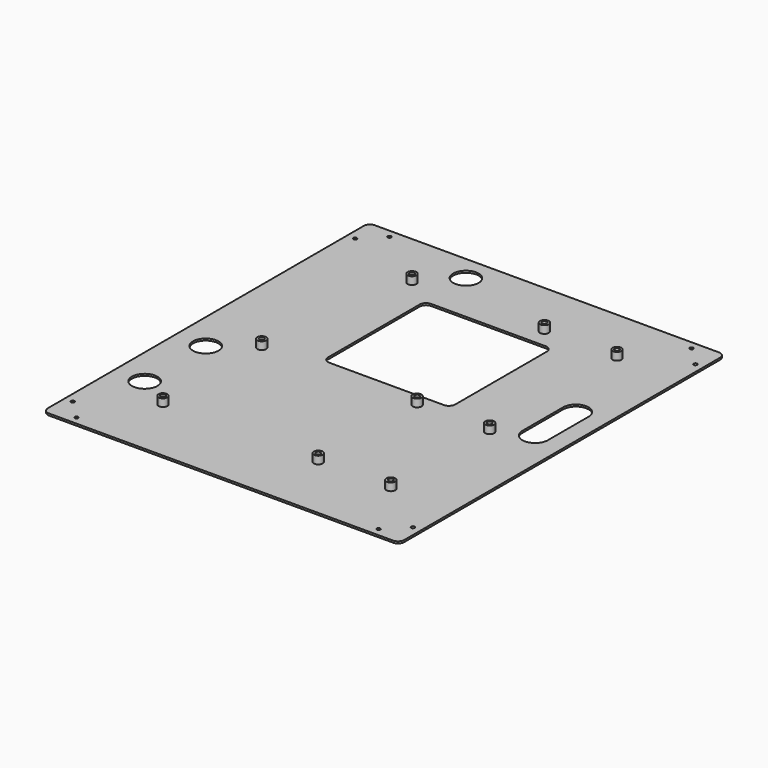
from build123d import *

# Parameters (mm, degrees)
F0_R     = 1.7526
F0_R_2   = 12.7
F0_R_3   = 4.445
F1_DEPTH = 1.905
F0_R_4   = 2.3876
F2_DEPTH = 9.525


# Not quite as in the source:
# - a feature names something its author has since deleted; it is built from what else it names


with BuildPart() as f1:
    # F0 (on Top) → F1 (new body)
    with BuildSketch(Plane.XY):
        with BuildLine():
            Line((192.8597838237, 278.8835931593), (-150.0402161763, 278.8835931593))
            ThreePointArc((-150.0402161763, 278.8835931593), (-154.5303442368, 277.0237212199), (-156.3902161763, 272.5335931593))
            Line((-156.3902161763, 272.5335931593), (-156.3902161763, -121.1664068407))
            ThreePointArc((-156.3902161763, -121.1664068407), (-154.5303442368, -125.6565349012), (-150.0402161763, -127.5164068407))
            Line((-150.0402161763, -127.5164068407), (192.8597838237, -127.5164068407))
            ThreePointArc((192.8597838237, -127.5164068407), (197.3499118843, -125.6565349012), (199.2097838237, -121.1664068407))
            Line((199.2097838237, -121.1664068407), (199.2097838237, 272.5335931593))
            ThreePointArc((199.2097838237, 272.5335931593), (197.3499118843, 277.0237212199), (192.8597838237, 278.8835931593))
        make_face()
        with Locations((-129.2376161763, -119.4138068407)):
            Circle(F0_R, mode=Mode.SUBTRACT)
        with Locations((-148.2876161763, -100.3638068407)):
            Circle(F0_R, mode=Mode.SUBTRACT)
        with Locations((-125.9102161763, -38.6164068407)):
            Circle(F0_R_2, mode=Mode.SUBTRACT)
        with Locations((-125.9102161763, 37.5835931593)):
            Circle(F0_R_2, mode=Mode.SUBTRACT)
        with Locations((172.0571838237, -119.4138068407)):
            Circle(F0_R, mode=Mode.SUBTRACT)
        with Locations((191.1071838237, -100.3638068407)):
            Circle(F0_R, mode=Mode.SUBTRACT)
        with Locations((-148.2876161763, 251.7309931593)):
            Circle(F0_R, mode=Mode.SUBTRACT)
        with Locations((-129.2376161763, 270.7809931593)):
            Circle(F0_R, mode=Mode.SUBTRACT)
        with Locations((-39.1178902483, 253.4835931593)):
            Circle(F0_R_2, mode=Mode.SUBTRACT)
        Polygon((64.5897838237, -76.7164068407), (-100.5102161763, -76.7164068407), (-100.5102161763, 140.7156608748), (-100.5102161763, 228.0835931593), (143.3297838237, 228.0835931593), (143.3297838237, -76.7164068407), align=None, mode=Mode.SUBTRACT)
        with BuildLine():
            Line((156.0297838237, 79.9791118101), (156.0297838237, 130.7791118101))
            ThreePointArc((156.0297838237, 130.7791118101), (168.7297838237, 143.4791118101), (181.4297838237, 130.7791118101))
            Line((181.4297838237, 130.7791118101), (181.4297838237, 79.9791118101))
            ThreePointArc((181.4297838237, 79.9791118101), (168.7297838237, 67.2791118101), (156.0297838237, 79.9791118101))
        make_face(mode=Mode.SUBTRACT)
        with Locations((191.1071838237, 251.7309931593)):
            Circle(F0_R, mode=Mode.SUBTRACT)
        with Locations((172.0571838237, 270.7809931593)):
            Circle(F0_R, mode=Mode.SUBTRACT)
        Polygon((-100.5102161763, 140.7156608748), (-100.5102161763, -76.7164068407), (64.5897838237, -76.7164068407), (143.3297838237, -76.7164068407), (143.3297838237, 228.0835931593), (-100.5102161763, 228.0835931593), align=None)
        with Locations((-90.3502161763, -60.2064068407)):
            Circle(F0_R_3, mode=Mode.SUBTRACT)
        with Locations((-90.3502161763, 62.9835931593)):
            Circle(F0_R_3, mode=Mode.SUBTRACT)
        with Locations((64.5897838237, -60.2064068407)):
            Circle(F0_R_3, mode=Mode.SUBTRACT)
        with Locations((136.9797838237, -60.2064068407)):
            Circle(F0_R_3, mode=Mode.SUBTRACT)
        with Locations((64.5897838237, 62.9835931593)):
            Circle(F0_R_3, mode=Mode.SUBTRACT)
        with Locations((136.9797838237, 62.9835931593)):
            Circle(F0_R_3, mode=Mode.SUBTRACT)
        with Locations((-67.4902161763, 221.7335931593)):
            Circle(F0_R_3, mode=Mode.SUBTRACT)
        with BuildLine():
            Line((-33.2002161763, 202.6835931593), (81.0997838237, 202.6835931593))
            ThreePointArc((81.0997838237, 202.6835931593), (85.5899118843, 200.8237212199), (87.4497838237, 196.3335931593))
            Line((87.4497838237, 196.3335931593), (87.4497838237, 82.0335931593))
            ThreePointArc((87.4497838237, 82.0335931593), (85.5899118843, 77.5434650988), (81.0997838237, 75.6835931593))
            Line((81.0997838237, 75.6835931593), (-33.2002161763, 75.6835931593))
            ThreePointArc((-33.2002161763, 75.6835931593), (-37.6903442368, 77.5434650988), (-39.5502161763, 82.0335931593))
            Line((-39.5502161763, 82.0335931593), (-39.5502161763, 196.3335931593))
            ThreePointArc((-39.5502161763, 196.3335931593), (-37.6903442368, 200.8237212199), (-33.2002161763, 202.6835931593))
        make_face(mode=Mode.SUBTRACT)
        with Locations((64.5897838237, 221.7335931593)):
            Circle(F0_R_3, mode=Mode.SUBTRACT)
        with Locations((136.9797838237, 221.7335931593)):
            Circle(F0_R_3, mode=Mode.SUBTRACT)
    extrude(amount=F1_DEPTH)


with BuildPart() as f1b:
    # F0 (on Top) → F1, piece 2 (new body)
    with BuildSketch(Plane.XY):
        with Locations((64.5897838237, 62.9835931593)):
            Circle(F0_R_4)
    extrude(amount=F1_DEPTH)


with BuildPart() as f1c:
    # F0 (on Top) → F1, piece 3 (new body)
    with BuildSketch(Plane.XY):
        with Locations((-90.3502161763, 62.9835931593)):
            Circle(F0_R_4)
    extrude(amount=F1_DEPTH)


with BuildPart() as f1d:
    # F0 (on Top) → F1, piece 4 (new body)
    with BuildSketch(Plane.XY):
        with Locations((-90.3502161763, -60.2064068407)):
            Circle(F0_R_4)
    extrude(amount=F1_DEPTH)


with BuildPart() as f1e:
    # F0 (on Top) → F1, piece 5 (new body)
    with BuildSketch(Plane.XY):
        with Locations((64.5897838237, -60.2064068407)):
            Circle(F0_R_4)
    extrude(amount=F1_DEPTH)


with BuildPart() as f1f:
    # F0 (on Top) → F1, piece 6 (new body)
    with BuildSketch(Plane.XY):
        with Locations((136.9797838237, -60.2064068407)):
            Circle(F0_R_4)
    extrude(amount=F1_DEPTH)


with BuildPart() as f2:
    # F0 (on Top) → F2 (new body)
    with BuildSketch(Plane.XY):
        with Locations((-90.3502161763, -60.2064068407)):
            Circle(F0_R_3)
        with Locations((-90.3502161763, -60.2064068407)):
            Circle(F0_R_4, mode=Mode.SUBTRACT)
    extrude(amount=F2_DEPTH)


with BuildPart() as f2b:
    # F0 (on Top) → F2, piece 2 (new body)
    with BuildSketch(Plane.XY):
        with Locations((-90.3502161763, 62.9835931593)):
            Circle(F0_R_3)
        with Locations((-90.3502161763, 62.9835931593)):
            Circle(F0_R_4, mode=Mode.SUBTRACT)
    extrude(amount=F2_DEPTH)


with BuildPart() as f2c:
    # F0 (on Top) → F2, piece 3 (new body)
    with BuildSketch(Plane.XY):
        with Locations((64.5897838237, 62.9835931593)):
            Circle(F0_R_3)
        with Locations((64.5897838237, 62.9835931593)):
            Circle(F0_R_4, mode=Mode.SUBTRACT)
    extrude(amount=F2_DEPTH)


with BuildPart() as f2d:
    # F0 (on Top) → F2, piece 4 (new body)
    with BuildSketch(Plane.XY):
        with Locations((136.9797838237, 62.9835931593)):
            Circle(F0_R_3)
        with Locations((136.9797838237, 62.9835931593)):
            Circle(F0_R_4, mode=Mode.SUBTRACT)
    extrude(amount=F2_DEPTH)


with BuildPart() as f2e:
    # F0 (on Top) → F2, piece 5 (new body)
    with BuildSketch(Plane.XY):
        with Locations((64.5897838237, -60.2064068407)):
            Circle(F0_R_3)
        with Locations((64.5897838237, -60.2064068407)):
            Circle(F0_R_4, mode=Mode.SUBTRACT)
    extrude(amount=F2_DEPTH)


with BuildPart() as f2f:
    # F0 (on Top) → F2, piece 6 (new body)
    with BuildSketch(Plane.XY):
        with Locations((136.9797838237, -60.2064068407)):
            Circle(F0_R_3)
        with Locations((136.9797838237, -60.2064068407)):
            Circle(F0_R_4, mode=Mode.SUBTRACT)
    extrude(amount=F2_DEPTH)


with BuildPart() as f2g:
    # F0 (on Top) → F2, piece 7 (new body)
    with BuildSketch(Plane.XY):
        with Locations((136.9797838237, 221.7335931593)):
            Circle(F0_R_3)
        with Locations((136.9797838237, 221.7335931593)):
            Circle(F0_R_4, mode=Mode.SUBTRACT)
    extrude(amount=F2_DEPTH)


with BuildPart() as f2h:
    # F0 (on Top) → F2, piece 8 (new body)
    with BuildSketch(Plane.XY):
        with Locations((64.5897838237, 221.7335931593)):
            Circle(F0_R_3)
        with Locations((64.5897838237, 221.7335931593)):
            Circle(F0_R_4, mode=Mode.SUBTRACT)
    extrude(amount=F2_DEPTH)


with BuildPart() as f2i:
    # F0 (on Top) → F2, piece 9 (new body)
    with BuildSketch(Plane.XY):
        with Locations((-67.4902161763, 221.7335931593)):
            Circle(F0_R_3)
        with Locations((-67.4902161763, 221.7335931593)):
            Circle(F0_R_4, mode=Mode.SUBTRACT)
    extrude(amount=F2_DEPTH)


solid = Compound([f1.part, f1b.part, f1c.part, f1d.part, f1e.part, f1f.part, f2.part, f2b.part, f2c.part, f2d.part, f2e.part, f2f.part, f2g.part, f2h.part, f2i.part])
